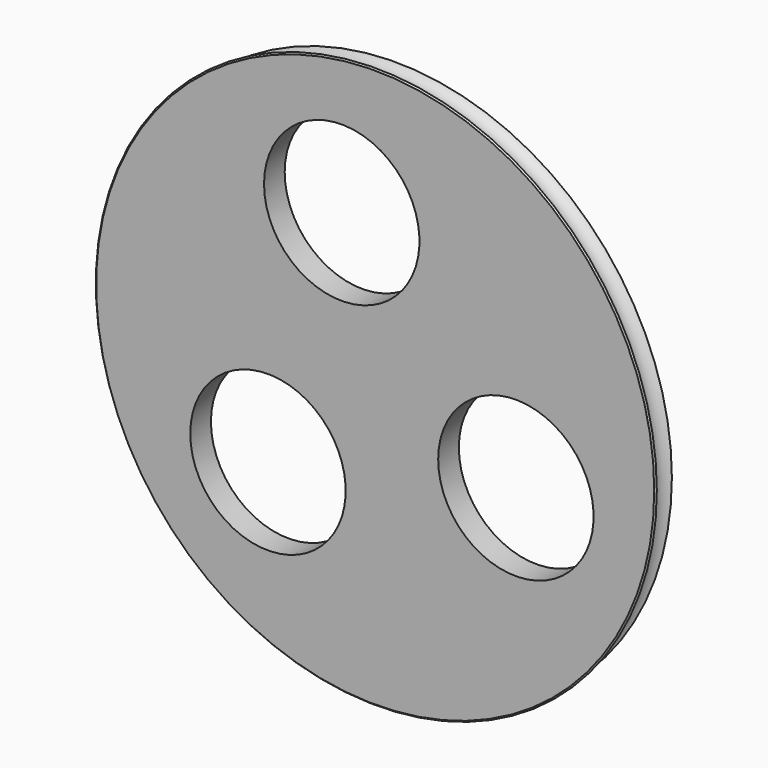
from build123d import *

# Parameters (mm, degrees)
F0_R     = 279.4
F1_DEPTH = 25.4
F2_R     = 13.3406236018
F6_R     = 76.3831689613
F7_DEPTH = 25.4


# Not quite as in the source:
# - a fillet or chamfer that OpenCascade refuses, or shapes differently, is made with other operations: its cross-section is extruded or revolved along the edge and cut away or added


with BuildPart() as f1:
    # F0 (on Front) → F1 (new body)
    with BuildSketch(Plane.XZ):
        Circle(F0_R)
    extrude(amount=F1_DEPTH)

    # F2 (on Top) → F3 (revolve, cut)
    with BuildSketch(Plane.XY):
        with Locations((278.8262367249, -11.0273361206)):
            Circle(F2_R)
    revolve(axis=Axis((0, 0, 0), (0, 1, 0)), mode=Mode.SUBTRACT)

    # F4: chamfer of 5.08 on 1 edges, made by hand

    # F4_s1 → F4_t2 (revolve, cut)
    with BuildSketch(Plane.XY):
        Polygon((279.4, -20.32), (274.32, -25.4), (279.4, -25.4), align=None)
    revolve(axis=Axis((0, -25.4, 0), (0, -1, 0)), mode=Mode.SUBTRACT)

    # F6 (on face) → F7 (cut)
    with BuildSketch(Plane(origin=(0, 0, 0), x_dir=(-1, 0, 0), z_dir=(0, 1, 0))):
        with Locations((-138.2894814014, -41.8609678745)):
            Circle(F6_R)
        with Locations((32.8920790944, 140.6926879071)):
            Circle(F6_R)
        with Locations((105.3974023071, -98.8317200326)):
            Circle(F6_R)
    extrude(amount=-F7_DEPTH, mode=Mode.SUBTRACT)


solid = f1.part
